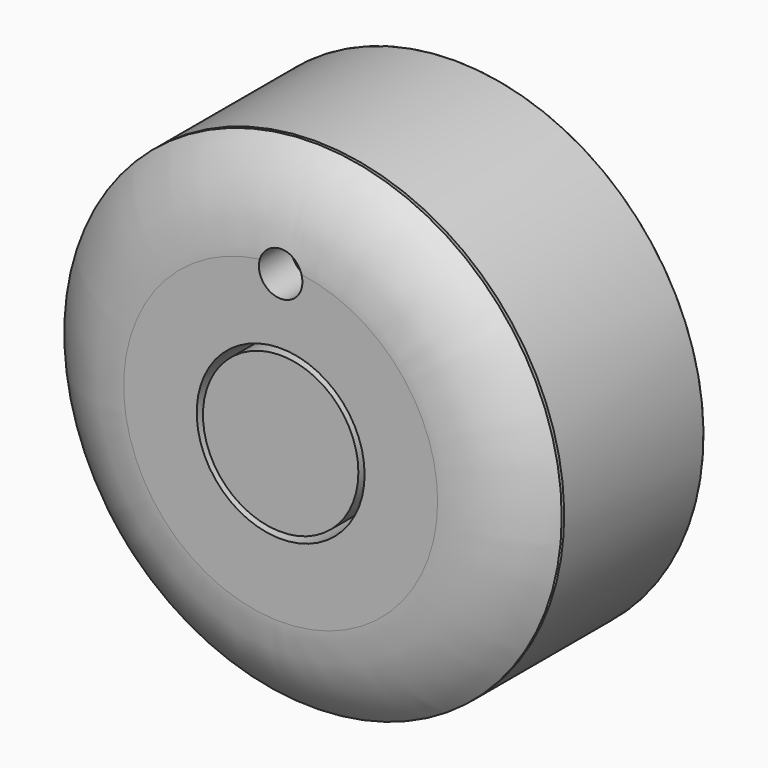
from build123d import *

# Parameters (mm, degrees)
F0_R     = 10.16
F0_R_2   = 3.429
F1_DEPTH = 10.414
F2_W     = 7.239
F2_H     = 5.588
F4_R     = 0.889
F5_DEPTH = 10.415
F6_W     = 7.112
F6_H     = 5.08
F8_R     = 3.175
F9_DEPTH = 9.525


# Not quite as in the source:
# - a fillet or chamfer that OpenCascade refuses, or shapes differently, is made with other operations: its cross-section is extruded or revolved along the edge and cut away or added


with BuildPart() as f1:
    # F0 (on Front) → F1 (new body)
    with BuildSketch(Plane.XZ):
        Circle(F0_R)
        Circle(F0_R_2, mode=Mode.SUBTRACT)
    extrude(amount=F1_DEPTH)

    # F2 (on Right) → F3 (revolve, cut)
    with BuildSketch(Plane.YZ):
        with Locations((-5.1435, 7.62)):
            Rectangle(F2_W, F2_H)
    revolve(axis=Axis((0, -10.414, 0), (0, -1, 0)), mode=Mode.SUBTRACT)

    # F4 (on face) → F5 (cut, through all)
    with BuildSketch(Plane(origin=(0, 0, 0), x_dir=(-1, 0, 0), z_dir=(0, 1, 0))):
        with Locations((0, 6.096)):
            Circle(F4_R)
    extrude(amount=-F5_DEPTH, mode=Mode.SUBTRACT)

    # F10: fillet of radius 5.08 on 2 edges, made by hand

    # F10_s1 → F10_t2 (revolve, cut)
    with BuildSketch(Plane.XY):
        with BuildLine():
            ThreePointArc((6.4118859409, -10.414), (8.459699409, -9.9829633253), (10.16, -8.763))
            Line((10.16, -8.763), (10.16, -10.414))
            Line((10.16, -10.414), (6.4118859409, -10.414))
        make_face()
    revolve(axis=Axis((0, -10.414, 0), (0, -1, 0)), mode=Mode.SUBTRACT)

    # F10_s3 → F10_t4 (revolve, cut)
    with BuildSketch(Plane.XY):
        with BuildLine():
            ThreePointArc((10.16, -1.524), (8.4996298982, -0.3964714157), (6.5321543583, 0))
            Line((6.5321543583, 0), (10.16, 0))
            Line((10.16, 0), (10.16, -1.524))
        make_face()
    revolve(axis=Axis((0, 0, 0), (0, -1, 0)), mode=Mode.SUBTRACT)


with BuildPart() as f7:
    # F6 (on Right) → F7 (revolve)
    with BuildSketch(Plane.YZ):
        with Locations((-5.08, 7.62)):
            Rectangle(F6_W, F6_H)
    revolve(axis=Axis((0, -10.414, 0), (0, -1, 0)))


with BuildPart() as f9:
    # F8 (on face) → F9 (new body)
    with BuildSketch(Plane.XZ.offset(10.414)):
        Circle(F8_R)
    extrude(amount=-F9_DEPTH)


solid = Compound([f1.part, f7.part, f9.part])
